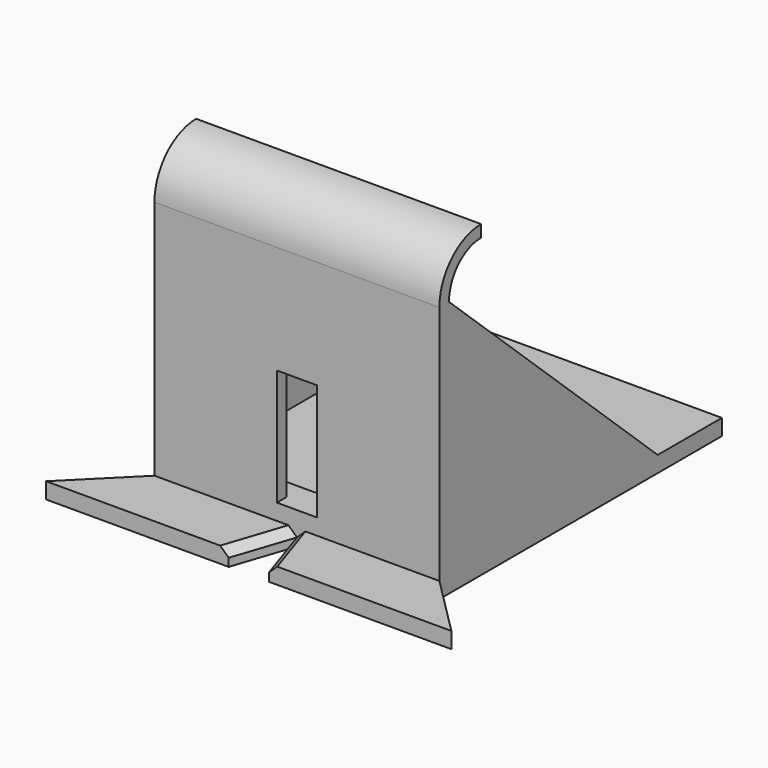
from build123d import *

# Parameters (mm, degrees)
F0_W         = 65
F0_H         = 65
F1_DEPTH     = 4
F3_DEPTH     = 60
F5_DEPTH     = 105.7
F7_DEPTH     = 25
F8_T4_DEPTH  = 26.0981202527
F8_T10_DEPTH = 26.0981202527
F9_SIZE      = 2
F10_DEPTH    = 20
F11_DEPTH    = 3
F12_DEPTH    = 3
F14_DEPTH    = 5
F15_DEPTH    = 15
F16_DEPTH    = 15
F18_DEPTH    = 71
F19_R        = 9.99999
F20_R        = 12.99999


# Not quite as in the source:
# - a fillet or chamfer that OpenCascade refuses, or shapes differently, is made with other operations: its cross-section is extruded or revolved along the edge and cut away or added
# - a fillet or chamfer is up to 0.001 mm smaller than in the source, because OpenCascade refuses the exact size


with BuildPart() as f1:
    # F0 (on Top) → F1 (new body)
    with BuildSketch(Plane.XY):
        Rectangle(F0_W, F0_H)
        Polygon((32.5, -32.5), (-32.5, -32.5), (-32.5, 32.5), (-35.5, 32.5), (-35.5, -35.5), (0, -35.5), (35.5, -35.5), (35.5, 32.5), (32.5, 32.5), align=None)
        Polygon((0, -35.5), (-35.5, -35.5), (-35.5, -50.5), (-5, -50.5), align=None)
        Polygon((-35.5, -50.5), (-35.5, -35.5), (-50.5, -50.5), align=None)
        Polygon((35.5, -50.5), (35.5, -35.5), (0, -35.5), (5, -50.5), (5.9827403165, -50.5), align=None)
        Polygon((50.5, -50.5), (35.5, -35.5), (35.5, -50.5), align=None)
    extrude(amount=F1_DEPTH)

    # F2 (on face) → F3 (join)
    with BuildSketch(Plane.XY.offset(4)):
        Polygon((32.5, -32.5), (-32.5, -32.5), (-32.5, 32.5), (-35.5, 32.5), (-35.5, -35.5), (0, -35.5), (35.5, -35.5), (35.5, 32.5), (32.5, 32.5), align=None)
    extrude(amount=F3_DEPTH)

    # F4 (on face) → F5 (cut)
    with BuildSketch(Plane.YZ.offset(35.5)):
        Polygon((-32.5, 64), (32.5, 4), (32.5, 64), align=None)
    extrude(amount=-F5_DEPTH, mode=Mode.SUBTRACT)

    # F6 (on face) → F7 (cut)
    with BuildSketch(Plane.XZ.offset(35.5)):
        Polygon((-5, 8), (0, 8), (3.482630942, 8), (25, 8), (25, 19), (5, 19), (5, 37), (0, 37), (-5, 37), (-5, 19), (-25, 19), (-25, 8), align=None)
    extrude(amount=-F7_DEPTH, mode=Mode.SUBTRACT)

    # F8: chamfer of 2 on 1 edges, made by hand


with BuildPart() as f8_tool2:
    # F8_s3 → F8_t4 (new body)
    with BuildSketch(Plane(origin=(-17.2764751324, -51.8294253971, 0), x_dir=(0, 0, 1), z_dir=(0.316227766, 0.9486832981, 0))):
        Polygon((2, 11.2260856936), (4, 9.2260856936), (4, 11.2260856936), align=None)
    extrude(amount=F8_T4_DEPTH)

    split(bisect_by=Plane.XZ.offset(35.5), keep=Keep.TOP)

    split(bisect_by=Plane(origin=(-10.65, -3.55, 0), x_dir=(0, 0, 1), z_dir=(-0.9486832981, -0.316227766, 0)), keep=Keep.TOP)


with BuildPart() as f1_1:
    add(f1.part)

    # F8_t1: cut F8_tool2
    add(f8_tool2.part, mode=Mode.SUBTRACT)


with BuildPart() as f8_tool8:
    # F8_s9 → F8_t10 (new body)
    with BuildSketch(Plane(origin=(-17.2764751324, -51.8294253971, 0), x_dir=(0, 0, 1), z_dir=(0.316227766, 0.9486832981, 0))):
        Polygon((2, 11.2260856936), (4, 9.2260856936), (4, 11.2260856936), align=None)
    extrude(amount=F8_T10_DEPTH)

    split(bisect_by=Plane.XZ.offset(32.5), keep=Keep.BOTTOM)

    split(bisect_by=Plane(origin=(-10.65, -3.55, 0), x_dir=(0, 0, 1), z_dir=(-0.9486832981, -0.316227766, 0)), keep=Keep.TOP)


with BuildPart() as f1_2:
    add(f1_1.part)

    # F8_t7: cut F8_tool8
    add(f8_tool8.part, mode=Mode.SUBTRACT)

    # F9
    f9_edges = [f1_2.edges().sort_by_distance(p)[0] for p in [
        (2.5, -43, 4),
    ]]
    chamfer(f9_edges, length=F9_SIZE)

    # F10 (add): a face of the model
    f10_faces = [f1_2.faces().sort_by_distance(p)[0] for p in [
        (0, 32.5, 2),
    ]]
    extrude(f10_faces, amount=F10_DEPTH)

    # F11 (add): a face of the model
    f11_faces = [f1_2.faces().sort_by_distance(p)[0] for p in [
        (15, -34, 19),
    ]]
    extrude(f11_faces, amount=-F11_DEPTH)

    # F12 (add): a face of the model
    f12_faces = [f1_2.faces().sort_by_distance(p)[0] for p in [
        (-15, -34, 19),
    ]]
    extrude(f12_faces, amount=-F12_DEPTH)

    # F13 (on face) → F14 (join)
    with BuildSketch(Plane(origin=(0, -32.5, 0), x_dir=(-1, 0, 0), z_dir=(0, 1, 0))):
        Polygon((32.5, 8), (25, 8), (-25, 8), (-32.5, 8), (-32.5, 4), (1, 4), (1, 3.8973665961), (1.1081851068, 4), (32.5, 4), align=None)
    extrude(amount=F14_DEPTH)

    # F15 (add): a face of the model
    f15_faces = [f1_2.faces().sort_by_distance(p)[0] for p in [
        (15, -34, 19),
    ]]
    extrude(f15_faces, amount=F15_DEPTH)

    # F16 (add): a face of the model
    f16_faces = [f1_2.faces().sort_by_distance(p)[0] for p in [
        (-15, -34, 19),
    ]]
    extrude(f16_faces, amount=F16_DEPTH)

    # F17 (on face) → F18 (join)
    with BuildSketch(Plane(origin=(-35.5, 0, 0), x_dir=(0, -1, 0), z_dir=(-1, 0, 0))):
        Polygon((32.5, 74), (32.5, 64), (35.5, 64), (35.5, 77), (22.5, 77), (22.5, 74), align=None)
    extrude(amount=-F18_DEPTH)

    # F19 (radius 10 in the source; OpenCascade refuses exactly that, so slightly less here)
    f19_edges = [f1_2.edges().sort_by_distance(p)[0] for p in [
        (0, -32.5, 74),
    ]]
    fillet(f19_edges, radius=F19_R)

    # F20 (radius 13 in the source; OpenCascade refuses exactly that, so slightly less here)
    f20_edges = [f1_2.edges().sort_by_distance(p)[0] for p in [
        (0, -35.5, 77),
    ]]
    fillet(f20_edges, radius=F20_R)


solid = f1_2.part
